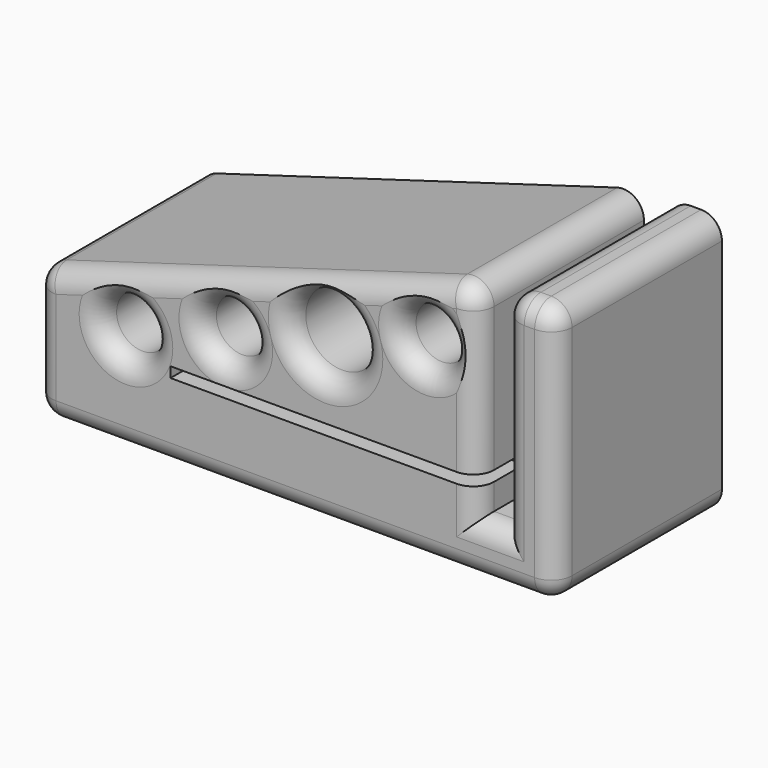
from build123d import *

# Parameters (mm, degrees)
F0_W          = 63.5
F0_H          = 25.4
F1_DEPTH      = 50.8
F2_W          = 3.175
F2_H          = 25.4
F3_DEPTH      = 25.4
F4_W          = 40.64
F4_H          = 1.27
F5_DEPTH      = 7.112
F6_W          = 63.5
F6_H          = 19.05
F7_DEPTH      = 25.4
F9_DEPTH      = 25.4
F10_W         = 37.465
F10_H         = 0.508
F11_DEPTH     = 11.938
F12_R         = 3.175
F12_R_2       = 4.445
F13_DEPTH     = 25.4
F14_T1_DEPTH  = 27.6113109813
F14_T3_DEPTH  = 31.3466050989
F14_T5_DEPTH  = 29.21
F14_T7_DEPTH  = 26.67
F14_T9_DEPTH  = 22.86
F14_T11_DEPTH = 9.525
F14_T13_DEPTH = 50.9659769086
F14_T15_DEPTH = 3.175
F14_T17_DEPTH = 58.42
F14_T19_DEPTH = 11.4344756075
F14_T21_DEPTH = 1.27
F14_T26_DEPTH = 2.54
F14_T32_DEPTH = 2.54
F14_S37_W     = 2.54
F14_S37_H     = 2.54
F14_T38_DEPTH = 2.54
F14_S43_W     = 2.54
F14_S43_H     = 2.54
F14_T44_DEPTH = 2.54
F14_S49_W     = 2.54
F14_S49_H     = 2.54
F14_T50_DEPTH = 2.54
F14_S55_W     = 2.54
F14_S55_H     = 2.54
F14_T56_DEPTH = 2.54
F14_T62_DEPTH = 23.9103579604
F14_T76_DEPTH = 29.21
F14_T80_DEPTH = 9.525
F14_T87_DEPTH = 15.875
F14_T91_DEPTH = 9.525


# Not quite as in the source:
# - a fillet or chamfer that OpenCascade refuses, or shapes differently, is made with other operations: its cross-section is extruded or revolved along the edge and cut away or added


with BuildPart() as f1:
    # F0 (on Top) → F1 (new body)
    with BuildSketch(Plane.XY):
        Rectangle(F0_W, F0_H)
    extrude(amount=F1_DEPTH)

    # F2 (on face) → F3 (cut)
    with BuildSketch(Plane.XY.offset(50.8)):
        with Locations((23.8125, 0)):
            Rectangle(F2_W, F2_H)
    extrude(amount=-F3_DEPTH, mode=Mode.SUBTRACT)

    # F4 (on face) → F5 (cut)
    with BuildSketch(Plane.XZ.offset(12.7)):
        with Locations((5.08, 29.21)):
            Rectangle(F4_W, F4_H)
    extrude(amount=-F5_DEPTH, mode=Mode.SUBTRACT)

    # F6 (on face) → F7 (cut)
    with BuildSketch(Plane.XZ.offset(12.7)):
        with Locations((0, 9.525)):
            Rectangle(F6_W, F6_H)
    extrude(amount=-F7_DEPTH, mode=Mode.SUBTRACT)

    # F8 (on face) → F9 (cut)
    with BuildSketch(Plane.XZ.offset(12.7)):
        Polygon((-31.75, 50.8), (-31.75, 34.925), (22.225, 50.8), align=None)
    extrude(amount=-F9_DEPTH, mode=Mode.SUBTRACT)

    # F10 (on face) → F11 (cut)
    with BuildSketch(Plane.XZ.offset(5.588)):
        with Locations((3.4925, 29.21)):
            Rectangle(F10_W, F10_H)
    extrude(amount=-F11_DEPTH, mode=Mode.SUBTRACT)

    # F12 (on face) → F13 (cut)
    with BuildSketch(Plane.XZ.offset(12.7)):
        with Locations((15.875, 42.5823529412)):
            Circle(F12_R)
        with Locations((3.69105813, 38.9988406265)):
            Circle(F12_R_2)
        with Locations((-8.4928837399, 35.4153283118)):
            Circle(F12_R)
        with Locations((-20.6768256099, 31.8318159971)):
            Circle(F12_R)
    extrude(amount=-F13_DEPTH, mode=Mode.SUBTRACT)

    # F14: fillet of radius 2.54 on 19 edges, made by hand

    # F14_s2 → F14_t1 (cut)
    with BuildSketch(Plane.XZ.offset(-17.4513109813)):
        with BuildLine():
            ThreePointArc((-31.75, 33.0244756075), (-31.2437187927, 34.5461811875), (-29.9267024629, 35.4612639815))
            Line((-29.9267024629, 35.4612639815), (-31.75, 34.925))
            Line((-31.75, 34.925), (-31.75, 33.0244756075))
        make_face()
    extrude(amount=F14_T1_DEPTH, mode=Mode.SUBTRACT)

    # F14_s4 → F14_t3 (cut)
    with BuildSketch(Plane.XZ.offset(-21.1866050989)):
        with BuildLine():
            ThreePointArc((18.9682975371, 49.8421463344), (21.20670558, 49.4390767532), (22.225, 47.4053579604))
            Line((22.225, 47.4053579604), (22.225, 50.8))
            Line((22.225, 50.8), (18.9682975371, 49.8421463344))
        make_face()
    extrude(amount=F14_T3_DEPTH, mode=Mode.SUBTRACT)

    # F14_s6 → F14_t5 (cut)
    with BuildSketch(Plane.XZ.offset(-19.05)):
        with BuildLine():
            ThreePointArc((27.94, 50.8), (26.1439487758, 50.0560512242), (25.4, 48.26))
            Line((25.4, 48.26), (25.4, 50.8))
            Line((25.4, 50.8), (27.94, 50.8))
        make_face()
        with BuildLine():
            ThreePointArc((31.75, 48.26), (31.0060512242, 50.0560512242), (29.21, 50.8))
            Line((29.21, 50.8), (31.75, 50.8))
            Line((31.75, 50.8), (31.75, 48.26))
        make_face()
        with BuildLine():
            ThreePointArc((-29.21, 19.05), (-31.0060512242, 19.7939487758), (-31.75, 21.59))
            Line((-31.75, 21.59), (-31.75, 19.05))
            Line((-31.75, 19.05), (-29.21, 19.05))
        make_face()
        with BuildLine():
            ThreePointArc((29.21, 19.05), (31.0060512242, 19.7939487758), (31.75, 21.59))
            Line((31.75, 21.59), (31.75, 19.05))
            Line((31.75, 19.05), (29.21, 19.05))
        make_face()
    extrude(amount=F14_T5_DEPTH, mode=Mode.SUBTRACT)

    # F14_s8 → F14_t7 (cut)
    with BuildSketch(Plane.XY.offset(21.59)):
        with BuildLine():
            ThreePointArc((31.75, -10.16), (31.0060512242, -11.9560512242), (29.21, -12.7))
            Line((29.21, -12.7), (31.75, -12.7))
            Line((31.75, -12.7), (31.75, -10.16))
        make_face()
    extrude(amount=F14_T7_DEPTH, mode=Mode.SUBTRACT)

    # F14_s10 → F14_t9 (cut)
    with BuildSketch(Plane.XY.offset(25.4)):
        with BuildLine():
            ThreePointArc((25.4, -10.16), (26.1439487758, -11.9560512242), (27.94, -12.7))
            Line((27.94, -12.7), (25.4, -12.7))
            Line((25.4, -12.7), (25.4, -10.16))
        make_face()
    extrude(amount=F14_T9_DEPTH, mode=Mode.SUBTRACT)

    # F14_s12 → F14_t11 (cut)
    with BuildSketch(Plane.XY.offset(25.4)):
        with BuildLine():
            ThreePointArc((22.225, -10.16), (21.4810512242, -11.9560512242), (19.685, -12.7))
            Line((19.685, -12.7), (22.225, -12.7))
            Line((22.225, -12.7), (22.225, -10.16))
        make_face()
    extrude(amount=F14_T11_DEPTH, mode=Mode.SUBTRACT)

    # F14_s14 → F14_t13 (cut)
    with BuildSketch(Plane(origin=(-17.9446164757, 0, -5.2778283752), x_dir=(0, 1, 0), z_dir=(0.9593655016, 0, 0.282166324))):
        with BuildLine():
            ThreePointArc((-10.16, 42.4646209291), (-11.9560512242, 41.7206721533), (-12.7, 39.9246209291))
            Line((-12.7, 39.9246209291), (-12.7, 42.4646209291))
            Line((-12.7, 42.4646209291), (-10.16, 42.4646209291))
        make_face()
    extrude(amount=F14_T13_DEPTH, mode=Mode.SUBTRACT)

    # F14_s16 → F14_t15 (cut)
    with BuildSketch(Plane.YZ.offset(22.225)):
        with BuildLine():
            ThreePointArc((-10.16, 25.4), (-11.9560512242, 24.6560512242), (-12.7, 22.86))
            Line((-12.7, 22.86), (-12.7, 25.4))
            Line((-12.7, 25.4), (-10.16, 25.4))
        make_face()
    extrude(amount=F14_T15_DEPTH, mode=Mode.SUBTRACT)

    # F14_s18 → F14_t17 (cut)
    with BuildSketch(Plane.YZ.offset(-29.21)):
        with BuildLine():
            ThreePointArc((-10.16, 19.05), (-11.9560512242, 19.7939487758), (-12.7, 21.59))
            Line((-12.7, 21.59), (-12.7, 19.05))
            Line((-12.7, 19.05), (-10.16, 19.05))
        make_face()
    extrude(amount=F14_T17_DEPTH, mode=Mode.SUBTRACT)

    # F14_s20 → F14_t19 (cut)
    with BuildSketch(Plane.XY.offset(21.59)):
        with BuildLine():
            ThreePointArc((-31.75, -10.16), (-31.0060512242, -11.9560512242), (-29.21, -12.7))
            Line((-29.21, -12.7), (-31.75, -12.7))
            Line((-31.75, -12.7), (-31.75, -10.16))
        make_face()
    extrude(amount=F14_T19_DEPTH, mode=Mode.SUBTRACT)

    # F14_s22 → F14_t21 (cut)
    with BuildSketch(Plane.YZ.offset(27.94)):
        with BuildLine():
            ThreePointArc((-10.16, 50.8), (-11.9560512242, 50.0560512242), (-12.7, 48.26))
            Line((-12.7, 48.26), (-12.7, 50.8))
            Line((-12.7, 50.8), (-10.16, 50.8))
        make_face()
    extrude(amount=F14_T21_DEPTH, mode=Mode.SUBTRACT)


with BuildPart() as f14_tool24:
    # F14_s25 → F14_t26 (new body)
    with BuildSketch(Plane.XZ.offset(10.16)):
        Polygon((-29.21, 33.0244756075), (-31.75, 33.0244756075), (-31.75, 34.925), (-29.9267024629, 35.4612639815), align=None)
    extrude(amount=F14_T26_DEPTH)

    # F14_s27 → F14_t28 (revolve, cut)
    with BuildSketch(Plane(origin=(-29.21, -10.16, 33.0244756075), x_dir=(0.8006766901, 0, -0.599096685), z_dir=(-0.599096685, 0, -0.8006766901))):
        with BuildLine():
            ThreePointArc((0, -2.54), (2.54, 0), (0, 2.54))
            Line((0, 2.54), (0, -2.54))
        make_face()
    revolve(axis=Axis((-29.21, -10.16, 33.0244756075), (0, -1, 0)), mode=Mode.SUBTRACT)


with BuildPart() as f1_1:
    add(f1.part)

    # F14_t23: cut F14_tool24
    add(f14_tool24.part, mode=Mode.SUBTRACT)


with BuildPart() as f14_tool30:
    # F14_s31 → F14_t32 (new body)
    with BuildSketch(Plane.XZ.offset(10.16)):
        Polygon((19.685, 47.4053579604), (18.9682975371, 49.8421463344), (22.225, 50.8), (22.225, 47.4053579604), align=None)
    extrude(amount=F14_T32_DEPTH)

    # F14_s33 → F14_t34 (revolve, cut)
    with BuildSketch(Plane(origin=(19.685, -10.16, 47.4053579604), x_dir=(-0.599096685, 0, -0.8006766901), z_dir=(-0.8006766901, 0, 0.599096685))):
        with BuildLine():
            ThreePointArc((0, -2.54), (2.54, 0), (0, 2.54))
            Line((0, 2.54), (0, -2.54))
        make_face()
    revolve(axis=Axis((19.685, -10.16, 47.4053579604), (0, -1, 0)), mode=Mode.SUBTRACT)


with BuildPart() as f1_2:
    add(f1_1.part)

    # F14_t29: cut F14_tool30
    add(f14_tool30.part, mode=Mode.SUBTRACT)


with BuildPart() as f14_tool36:
    # F14_s37 → F14_t38 (new body)
    with BuildSketch(Plane.XY.offset(48.26)):
        with Locations((26.67, -11.43)):
            Rectangle(F14_S37_W, F14_S37_H)
    extrude(amount=F14_T38_DEPTH)

    # F14_s39 → F14_t40 (revolve, cut)
    with BuildSketch(Plane(origin=(27.94, -10.16, 48.26), x_dir=(0.7071067812, 0.7071067812, 0), z_dir=(0.7071067812, -0.7071067812, 0))):
        with BuildLine():
            ThreePointArc((0, -2.54), (2.54, 0), (0, 2.54))
            Line((0, 2.54), (0, -2.54))
        make_face()
    revolve(axis=Axis((27.94, -10.16, 48.26), (0, 0, 1)), mode=Mode.SUBTRACT)


with BuildPart() as f1_3:
    add(f1_2.part)

    # F14_t35: cut F14_tool36
    add(f14_tool36.part, mode=Mode.SUBTRACT)


with BuildPart() as f14_tool42:
    # F14_s43 → F14_t44 (new body)
    with BuildSketch(Plane.XY.offset(21.59)):
        with Locations((30.48, -11.43)):
            Rectangle(F14_S43_W, F14_S43_H)
    extrude(amount=-F14_T44_DEPTH)

    # F14_s45 → F14_t46 (revolve, cut)
    with BuildSketch(Plane(origin=(29.21, -10.16, 21.59), x_dir=(-0.7071067812, 0.7071067812, 0), z_dir=(-0.7071067812, -0.7071067812, 0))):
        with BuildLine():
            ThreePointArc((0, -2.54), (2.54, 0), (0, 2.54))
            Line((0, 2.54), (0, -2.54))
        make_face()
    revolve(axis=Axis((29.21, -10.16, 21.59), (0, 0, -1)), mode=Mode.SUBTRACT)


with BuildPart() as f1_4:
    add(f1_3.part)

    # F14_t41: cut F14_tool42
    add(f14_tool42.part, mode=Mode.SUBTRACT)


with BuildPart() as f14_tool48:
    # F14_s49 → F14_t50 (new body)
    with BuildSketch(Plane.YZ.offset(29.21)):
        with Locations((-11.43, 49.53)):
            Rectangle(F14_S49_W, F14_S49_H)
    extrude(amount=F14_T50_DEPTH)

    # F14_s51 → F14_t52 (revolve, cut)
    with BuildSketch(Plane(origin=(29.21, -10.16, 48.26), x_dir=(0, 0.7071067812, -0.7071067812), z_dir=(0, -0.7071067812, -0.7071067812))):
        with BuildLine():
            ThreePointArc((0, -2.54), (2.54, 0), (0, 2.54))
            Line((0, 2.54), (0, -2.54))
        make_face()
    revolve(axis=Axis((29.21, -10.16, 48.26), (1, 0, 0)), mode=Mode.SUBTRACT)


with BuildPart() as f1_5:
    add(f1_4.part)

    # F14_t47: cut F14_tool48
    add(f14_tool48.part, mode=Mode.SUBTRACT)


with BuildPart() as f14_tool54:
    # F14_s55 → F14_t56 (new body)
    with BuildSketch(Plane.XY.offset(21.59)):
        with Locations((-30.48, -11.43)):
            Rectangle(F14_S55_W, F14_S55_H)
    extrude(amount=-F14_T56_DEPTH)

    # F14_s57 → F14_t58 (revolve, cut)
    with BuildSketch(Plane(origin=(-29.21, -10.16, 21.59), x_dir=(0.7071067812, 0.7071067812, 0), z_dir=(-0.7071067812, 0.7071067812, 0))):
        with BuildLine():
            ThreePointArc((0, -2.54), (2.54, 0), (0, 2.54))
            Line((0, 2.54), (0, -2.54))
        make_face()
    revolve(axis=Axis((-29.21, -10.16, 21.59), (0, 0, -1)), mode=Mode.SUBTRACT)


with BuildPart() as f1_6:
    add(f1_5.part)

    # F14_t53: cut F14_tool54
    add(f14_tool54.part, mode=Mode.SUBTRACT)


with BuildPart() as f14_tool60:
    # F14_s61 → F14_t62 (new body)
    with BuildSketch(Plane.XY.offset(47.4053579604)):
        with BuildLine():
            ThreePointArc((22.225, -10.16), (21.4810512242, -11.9560512242), (19.685, -12.7))
            Line((19.685, -12.7), (22.225, -12.7))
            Line((22.225, -12.7), (22.225, -10.16))
        make_face()
    extrude(amount=-F14_T62_DEPTH)

    split(bisect_by=Plane.XY.offset(25.4), keep=Keep.TOP)


with BuildPart() as f1_7:
    add(f1_6.part)

    # F14_t59: cut F14_tool60
    add(f14_tool60.part, mode=Mode.SUBTRACT)

    # F14_s64 → F14_t65 (revolve, cut)
    with BuildSketch(Plane.XY.offset(31.8318159971)):
        with BuildLine():
            ThreePointArc((-17.5018256099, -10.16), (-16.7578768341, -11.9560512242), (-14.9618256099, -12.7))
            Line((-14.9618256099, -12.7), (-17.5018256099, -12.7))
            Line((-17.5018256099, -12.7), (-17.5018256099, -10.16))
        make_face()
    revolve(axis=Axis((-20.6768256099, -12.7, 31.8318159971), (0, -1, 0)), mode=Mode.SUBTRACT)

    # F14_s66 → F14_t67 (revolve, cut)
    with BuildSketch(Plane.XY.offset(35.4153283118)):
        with BuildLine():
            ThreePointArc((-5.3178837399, -10.16), (-4.5739349641, -11.9560512242), (-2.7778837399, -12.7))
            Line((-2.7778837399, -12.7), (-5.3178837399, -12.7))
            Line((-5.3178837399, -12.7), (-5.3178837399, -10.16))
        make_face()
    revolve(axis=Axis((-8.4928837399, -12.7, 35.4153283118), (0, -1, 0)), mode=Mode.SUBTRACT)

    # F14_s68 → F14_t69 (revolve, cut)
    with BuildSketch(Plane.XY.offset(38.9988406265)):
        with BuildLine():
            ThreePointArc((8.13605813, -10.16), (8.8800069058, -11.9560512242), (10.67605813, -12.7))
            Line((10.67605813, -12.7), (8.13605813, -12.7))
            Line((8.13605813, -12.7), (8.13605813, -10.16))
        make_face()
    revolve(axis=Axis((3.69105813, -12.7, 38.9988406265), (0, -1, 0)), mode=Mode.SUBTRACT)

    # F14_s70 → F14_t71 (revolve, cut)
    with BuildSketch(Plane.XY.offset(42.5823529412)):
        with BuildLine():
            ThreePointArc((19.05, -10.16), (19.7939487758, -11.9560512242), (21.59, -12.7))
            Line((21.59, -12.7), (19.05, -12.7))
            Line((19.05, -12.7), (19.05, -10.16))
        make_face()
    revolve(axis=Axis((15.875, -12.7, 42.5823529412), (0, -1, 0)), mode=Mode.SUBTRACT)


with BuildPart() as f14_tool74:
    # F14_s75 → F14_t76 (new body)
    with BuildSketch(Plane.XY.offset(19.05)):
        with BuildLine():
            ThreePointArc((25.4, -10.16), (26.1439487758, -11.9560512242), (27.94, -12.7))
            Line((27.94, -12.7), (25.4, -12.7))
            Line((25.4, -12.7), (25.4, -10.16))
        make_face()
    extrude(amount=F14_T76_DEPTH)

    split(bisect_by=Plane.XY.offset(25.4), keep=Keep.BOTTOM)


with BuildPart() as f14_tool78:
    # F14_s79 → F14_t80 (new body)
    with BuildSketch(Plane.YZ.offset(22.225)):
        with BuildLine():
            ThreePointArc((-10.16, 25.4), (-11.9560512242, 24.6560512242), (-12.7, 22.86))
            Line((-12.7, 22.86), (-12.7, 25.4))
            Line((-12.7, 25.4), (-10.16, 25.4))
        make_face()
    extrude(amount=F14_T80_DEPTH)

    split(bisect_by=Plane.YZ.offset(25.4), keep=Keep.TOP)


with BuildPart() as f14_tool74_1:
    add(f14_tool74.part)

    # F14_t82: intersect F14_tool78
    add(f14_tool78.part, mode=Mode.INTERSECT)


with BuildPart() as f1_8:
    add(f1_7.part)

    # F14_t72: cut F14_tool74
    add(f14_tool74_1.part, mode=Mode.SUBTRACT)


with BuildPart() as f14_tool85:
    # F14_s86 → F14_t87 (new body)
    with BuildSketch(Plane.XY.offset(34.925)):
        with BuildLine():
            ThreePointArc((22.225, -10.16), (21.4810512242, -11.9560512242), (19.685, -12.7))
            Line((19.685, -12.7), (22.225, -12.7))
            Line((22.225, -12.7), (22.225, -10.16))
        make_face()
    extrude(amount=-F14_T87_DEPTH)

    split(bisect_by=Plane.XY.offset(25.4), keep=Keep.BOTTOM)


with BuildPart() as f14_tool89:
    # F14_s90 → F14_t91 (new body)
    with BuildSketch(Plane.YZ.offset(15.875)):
        with BuildLine():
            ThreePointArc((-10.16, 25.4), (-11.9560512242, 24.6560512242), (-12.7, 22.86))
            Line((-12.7, 22.86), (-12.7, 25.4))
            Line((-12.7, 25.4), (-10.16, 25.4))
        make_face()
    extrude(amount=F14_T91_DEPTH)

    split(bisect_by=Plane.YZ.offset(22.225), keep=Keep.BOTTOM)


with BuildPart() as f14_tool85_1:
    add(f14_tool85.part)

    # F14_t93: intersect F14_tool89
    add(f14_tool89.part, mode=Mode.INTERSECT)


with BuildPart() as f1_9:
    add(f1_8.part)

    # F14_t83: cut F14_tool85
    add(f14_tool85_1.part, mode=Mode.SUBTRACT)


solid = f1_9.part
